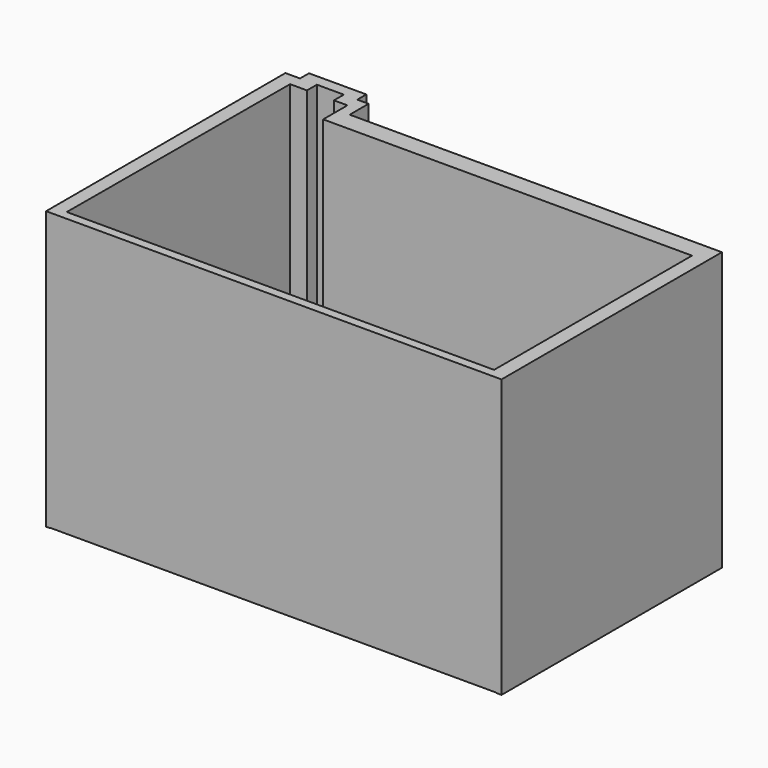
from build123d import *

# Parameters (mm, degrees)
F1_DEPTH      = 50
F2_DEPTH      = 25.4
F4_T1_DEPTH   = 7.325630635
F4_T3_DEPTH   = 9.8896528584
F4_T5_DEPTH   = 10.1948919696
F4_T7_DEPTH   = 14.7742944759
F4_T9_DEPTH   = 106.6527421576
F4_T11_DEPTH  = 67.1516433358
F4_T16_DEPTH  = 88.4586156969
F4_T22_DEPTH  = 17.6426691914
F4_T27_DEPTH  = 122.521271835
F4_T33_DEPTH  = 88.4586156969
F4_T38_DEPTH  = 122.521271835
F4_T47_DEPTH  = 88.4586156969
F4_T53_DEPTH  = 11.110594402
F4_T61_DEPTH  = 88.4586156969
F4_T66_DEPTH  = 11.110594402
F4_T74_DEPTH  = 13.8577054245
F4_T79_DEPTH  = 9.8896528584
F4_T87_DEPTH  = 9.8896528584
F4_T92_DEPTH  = 13.8577054245
F4_T100_DEPTH = 14.7742944759
F4_T105_DEPTH = 10.1948919696
F4_T113_DEPTH = 73.6837181253
F4_T118_DEPTH = 106.6527421576
F4_T126_DEPTH = 129.0533466244
F4_T132_DEPTH = 73.6837181253


# Not quite as in the source:
# - a fillet or chamfer that OpenCascade refuses, or shapes differently, is made with other operations: its cross-section is extruded or revolved along the edge and cut away or added
# - a feature of the source that left no trace in its solid (it failed there, or was rolled back) is left out


with BuildPart() as f1:
    # F0 (on Top) → F1 (new body)
    with BuildSketch(Plane.XY):
        Polygon((55.5458813906, -34.4724208117), (55.5458813906, 37.8682129085), (-45.4904846847, 37.8682129085), (-45.4904846847, 44.2790202796), (-48.5428348184, 44.2790202796), (-48.5428348184, 47.331366688), (-64.1098022461, 47.331366688), (-64.1098022461, 44.2790202796), (-68.0741816759, 44.2790202796), (-68.0741816759, 37.8682129085), (-68.0741816759, 32.6792225242), (-68.0741816759, -36.9142964482), (55.5458813906, -36.9142964482), align=None)
        Polygon((-48.5428348184, 32.6792225242), (51.5778325498, 32.6792225242), (51.5778325498, -34.4724208117), (-64.4113644958, -34.4724208117), (-64.1098022461, 40.9214422107), (-59.5312826335, 40.9214422107), (-59.5312826335, 44.2790202796), (-52.2056519985, 44.2790202796), (-52.2056519985, 40.9214422107), (-48.5428348184, 40.9214422107), align=None, mode=Mode.SUBTRACT)
    extrude(amount=F1_DEPTH)

    # F0 (on Top) + F1_face (on face) → F2 (join)
    with BuildSketch(Plane.XY):
        Polygon((55.5458813906, -34.4724208117), (55.5458813906, 37.8682129085), (-45.4904846847, 37.8682129085), (-45.4904846847, 44.2790202796), (-48.5428348184, 44.2790202796), (-48.5428348184, 47.331366688), (-64.1098022461, 47.331366688), (-64.1098022461, 44.2790202796), (-68.0741816759, 44.2790202796), (-68.0741816759, 37.8682129085), (-68.0741816759, 32.6792225242), (-68.0741816759, -36.9142964482), (55.5458813906, -36.9142964482), align=None)
        Polygon((-48.5428348184, 32.6792225242), (51.5778325498, 32.6792225242), (51.5778325498, -34.4724208117), (-64.4113644958, -34.4724208117), (-64.1098022461, 40.9214422107), (-59.5312826335, 40.9214422107), (-59.5312826335, 44.2790202796), (-52.2056519985, 44.2790202796), (-52.2056519985, 40.9214422107), (-48.5428348184, 40.9214422107), align=None, mode=Mode.SUBTRACT)
    with BuildSketch(Plane(origin=(-7.1792836418, 9.1982220042, 50), x_dir=(1, 0, 0), z_dir=(0, 0, 1))):
        Polygon((62.7251650324, -46.1125184524), (62.7251650324, 28.6699909043), (-38.3112010429, 28.6699909043), (-38.3112010429, 35.0807982755), (-41.3635511765, 35.0807982755), (-41.3635511765, 38.1331446838), (-56.9305186042, 38.1331446838), (-56.9305186042, 35.0807982755), (-60.8948980341, 35.0807982755), (-60.8948980341, -46.1125184524), align=None)
        Polygon((-56.9305186042, 31.7232202065), (-52.3519989917, 31.7232202065), (-52.3519989917, 35.0807982755), (-45.0263683567, 35.0807982755), (-45.0263683567, 31.7232202065), (-41.3635511765, 31.7232202065), (-41.3635511765, 23.48100052), (58.7571161917, 23.48100052), (58.7571161917, -43.6706428158), (-57.2320808539, -43.6706428158), align=None, mode=Mode.SUBTRACT)
    extrude(amount=F2_DEPTH)

    # F4: chamfer of 2.54 on 10 edges, made by hand

    # F4_s2 → F4_t1 (cut)
    with BuildSketch(Plane.YZ.offset(-59.5312826335)):
        Polygon((44.2790202796, 2.54), (46.8190202796, 0), (44.2790202796, 0), align=None)
    extrude(amount=F4_T1_DEPTH, mode=Mode.SUBTRACT)

    # F4_s4 → F4_t3 (cut)
    with BuildSketch(Plane.XZ.offset(-44.2790202796)):
        Polygon((-59.5312826335, 2.54), (-62.0712826335, 0), (-59.5312826335, 0), align=None)
        Polygon((-52.2056519985, 2.54), (-49.6656519985, 0), (-52.2056519985, 0), align=None)
    extrude(amount=F4_T3_DEPTH, mode=Mode.SUBTRACT)

    # F4_s6 → F4_t5 (cut)
    with BuildSketch(Plane.YZ.offset(-58.737726788)):
        Polygon((40.9214422107, 2.54), (43.4614422107, 0), (40.9214422107, 0), align=None)
    extrude(amount=F4_T5_DEPTH, mode=Mode.SUBTRACT)

    # F4_s8 → F4_t7 (cut)
    with BuildSketch(Plane.XZ.offset(-40.9214422107)):
        Polygon((-48.5428348184, 2.54), (-46.0028348184, 0), (-48.5428348184, 0), align=None)
    extrude(amount=F4_T7_DEPTH, mode=Mode.SUBTRACT)

    # F4_s10 → F4_t9 (cut)
    with BuildSketch(Plane.YZ.offset(-55.0749096078)):
        Polygon((32.6792225242, 2.54), (35.2192225242, 0), (32.6792225242, 0), align=None)
    extrude(amount=F4_T9_DEPTH, mode=Mode.SUBTRACT)

    # F4_s12 → F4_t11 (cut)
    with BuildSketch(Plane.XZ.offset(-32.6792225242)):
        Polygon((51.5778325498, 2.54), (54.1178325498, 0), (51.5778325498, 0), align=None)
    extrude(amount=F4_T11_DEPTH, mode=Mode.SUBTRACT)


with BuildPart() as f4_tool14:
    # F4_s15 → F4_t16 (new body)
    with BuildSketch(Plane(origin=(-0.1650388622, -41.2615219051, 0), x_dir=(0, 0, 1), z_dir=(0.0039997929, 0.9999920008, 0))):
        Polygon((2.54, -64.2729667124), (0, -66.8129667124), (0, -64.2729667124), align=None)
    extrude(amount=F4_T16_DEPTH)

    split(bisect_by=Plane.XZ.offset(34.4724208117), keep=Keep.BOTTOM)

    split(bisect_by=Plane.XZ.offset(-40.9214422107), keep=Keep.TOP)


with BuildPart() as f1_1:
    add(f1.part)

    # F4_t13: cut F4_tool14
    add(f4_tool14.part, mode=Mode.SUBTRACT)


with BuildPart() as f4_tool20:
    # F4_s21 → F4_t22 (new body)
    with BuildSketch(Plane.YZ.offset(-70.6418770355)):
        Polygon((40.9214422107, 2.54), (43.4614422107, 0), (40.9214422107, 0), align=None)
    extrude(amount=F4_T22_DEPTH)

    split(bisect_by=Plane(origin=(-64.2724525799, 0.2570785554, 0), x_dir=(0, 0, 1), z_dir=(0.9999920008, -0.0039997929, 0)), keep=Keep.TOP)


with BuildPart() as f1_2:
    add(f1_1.part)

    # F4_t19: cut F4_tool20
    add(f4_tool20.part, mode=Mode.SUBTRACT)


with BuildPart() as f4_tool25:
    # F4_s26 → F4_t27 (new body)
    with BuildSketch(Plane.YZ.offset(51.5778325498)):
        Polygon((-34.4724208117, 2.54), (-37.0124208117, 0), (-34.4724208117, 0), align=None)
    extrude(amount=-F4_T27_DEPTH)

    split(bisect_by=Plane(origin=(-64.2724525799, 0.2570785554, 0), x_dir=(0, 0, 1), z_dir=(0.9999920008, -0.0039997929, 0)), keep=Keep.TOP)


with BuildPart() as f1_3:
    add(f1_2.part)

    # F4_t24: cut F4_tool25
    add(f4_tool25.part, mode=Mode.SUBTRACT)


with BuildPart() as f4_tool31:
    # F4_s32 → F4_t33 (new body)
    with BuildSketch(Plane(origin=(-0.1650388622, -41.2615219051, 0), x_dir=(0, 0, 1), z_dir=(0.0039997929, 0.9999920008, 0))):
        Polygon((2.54, -64.2729667124), (0, -66.8129667124), (0, -64.2729667124), align=None)
    extrude(amount=F4_T33_DEPTH)

    split(bisect_by=Plane.XZ.offset(34.4724208117), keep=Keep.TOP)

    split(bisect_by=Plane.XZ.offset(36.9142964482), keep=Keep.BOTTOM)


with BuildPart() as f4_tool36:
    # F4_s37 → F4_t38 (new body)
    with BuildSketch(Plane.YZ.offset(51.5778325498)):
        Polygon((-34.4724208117, 2.54), (-37.0124208117, 0), (-34.4724208117, 0), align=None)
    extrude(amount=-F4_T38_DEPTH)

    split(bisect_by=Plane(origin=(-64.2724525799, 0.2570785554, 0), x_dir=(0, 0, 1), z_dir=(-0.9999920008, 0.0039997929, 0)), keep=Keep.TOP)

    split(bisect_by=Plane.YZ.offset(-68.0741816759), keep=Keep.TOP)

    split(bisect_by=Plane.XZ.offset(36.9142964482), keep=Keep.BOTTOM)


with BuildPart() as f4_tool31_1:
    add(f4_tool31.part)

    # F4_t42: intersect F4_tool36
    add(f4_tool36.part, mode=Mode.INTERSECT)


with BuildPart() as f1_4:
    add(f1_3.part)

    # F4_t29: cut F4_tool31
    add(f4_tool31_1.part, mode=Mode.SUBTRACT)


with BuildPart() as f4_tool45:
    # F4_s46 → F4_t47 (new body)
    with BuildSketch(Plane(origin=(-0.1650388622, -41.2615219051, 0), x_dir=(0, 0, 1), z_dir=(0.0039997929, 0.9999920008, 0))):
        Polygon((2.54, -64.2729667124), (0, -66.8129667124), (0, -64.2729667124), align=None)
    extrude(amount=F4_T47_DEPTH)

    split(bisect_by=Plane.XZ.offset(-40.9214422107), keep=Keep.BOTTOM)

    split(bisect_by=Plane.XZ.offset(-44.2790202796), keep=Keep.TOP)

    split(bisect_by=Plane.YZ.offset(-64.1098022461), keep=Keep.BOTTOM)


with BuildPart() as f4_tool51:
    # F4_s52 → F4_t53 (new body)
    with BuildSketch(Plane.YZ.offset(-70.6418770355)):
        Polygon((40.9214422107, 2.54), (43.4614422107, 0), (40.9214422107, 0), align=None)
    extrude(amount=F4_T53_DEPTH)

    split(bisect_by=Plane(origin=(-64.2724525799, 0.2570785554, 0), x_dir=(0, 0, 1), z_dir=(-0.9999920008, 0.0039997929, 0)), keep=Keep.TOP)

    split(bisect_by=Plane.YZ.offset(-68.0741816759), keep=Keep.TOP)


with BuildPart() as f4_tool45_1:
    add(f4_tool45.part)

    # F4_t56: intersect F4_tool51
    add(f4_tool51.part, mode=Mode.INTERSECT)


with BuildPart() as f1_5:
    add(f1_4.part)

    # F4_t43: cut F4_tool45
    add(f4_tool45_1.part, mode=Mode.SUBTRACT)


with BuildPart() as f4_tool59:
    # F4_s60 → F4_t61 (new body)
    with BuildSketch(Plane(origin=(-0.1650388622, -41.2615219051, 0), x_dir=(0, 0, 1), z_dir=(0.0039997929, 0.9999920008, 0))):
        Polygon((2.54, -64.2729667124), (0, -66.8129667124), (0, -64.2729667124), align=None)
    extrude(amount=F4_T61_DEPTH)

    split(bisect_by=Plane.XZ.offset(-44.2790202796), keep=Keep.TOP)

    split(bisect_by=Plane.YZ.offset(-64.1098022461), keep=Keep.TOP)


with BuildPart() as f4_tool64:
    # F4_s65 → F4_t66 (new body)
    with BuildSketch(Plane.YZ.offset(-70.6418770355)):
        Polygon((40.9214422107, 2.54), (43.4614422107, 0), (40.9214422107, 0), align=None)
    extrude(amount=F4_T66_DEPTH)

    split(bisect_by=Plane(origin=(-64.2724525799, 0.2570785554, 0), x_dir=(0, 0, 1), z_dir=(-0.9999920008, 0.0039997929, 0)), keep=Keep.TOP)

    split(bisect_by=Plane.YZ.offset(-68.0741816759), keep=Keep.TOP)


with BuildPart() as f4_tool59_1:
    add(f4_tool59.part)

    # F4_t69: intersect F4_tool64
    add(f4_tool64.part, mode=Mode.INTERSECT)


with BuildPart() as f1_6:
    add(f1_5.part)

    # F4_t57: cut F4_tool59
    add(f4_tool59_1.part, mode=Mode.SUBTRACT)


with BuildPart() as f4_tool72:
    # F4_s73 → F4_t74 (new body)
    with BuildSketch(Plane.YZ.offset(-66.063357423)):
        Polygon((44.2790202796, 2.54), (46.8190202796, 0), (44.2790202796, 0), align=None)
    extrude(amount=F4_T74_DEPTH)

    split(bisect_by=Plane.YZ.offset(-59.5312826335), keep=Keep.BOTTOM)

    split(bisect_by=Plane.YZ.offset(-64.1098022461), keep=Keep.TOP)


with BuildPart() as f4_tool77:
    # F4_s78 → F4_t79 (new body)
    with BuildSketch(Plane.XZ.offset(-40.9214422107)):
        Polygon((-59.5312826335, 2.54), (-62.0712826335, 0), (-59.5312826335, 0), align=None)
    extrude(amount=-F4_T79_DEPTH)

    split(bisect_by=Plane.XZ.offset(-44.2790202796), keep=Keep.BOTTOM)

    split(bisect_by=Plane.XZ.offset(-47.331366688), keep=Keep.TOP)


with BuildPart() as f4_tool72_1:
    add(f4_tool72.part)

    # F4_t82: intersect F4_tool77
    add(f4_tool77.part, mode=Mode.INTERSECT)


with BuildPart() as f1_7:
    add(f1_6.part)

    # F4_t70: cut F4_tool72
    add(f4_tool72_1.part, mode=Mode.SUBTRACT)


with BuildPart() as f4_tool85:
    # F4_s86 → F4_t87 (new body)
    with BuildSketch(Plane.XZ.offset(-50.8110950691)):
        Polygon((-52.2056519985, 2.54), (-49.6656519985, 0), (-52.2056519985, 0), align=None)
    extrude(amount=F4_T87_DEPTH)

    split(bisect_by=Plane.XZ.offset(-44.2790202796), keep=Keep.BOTTOM)

    split(bisect_by=Plane.XZ.offset(-47.331366688), keep=Keep.TOP)


with BuildPart() as f4_tool90:
    # F4_s91 → F4_t92 (new body)
    with BuildSketch(Plane.YZ.offset(-59.5312826335)):
        Polygon((44.2790202796, 2.54), (46.8190202796, 0), (44.2790202796, 0), align=None)
    extrude(amount=F4_T92_DEPTH)

    split(bisect_by=Plane.YZ.offset(-52.2056519985), keep=Keep.TOP)

    split(bisect_by=Plane.YZ.offset(-48.5428348184), keep=Keep.BOTTOM)


with BuildPart() as f4_tool85_1:
    add(f4_tool85.part)

    # F4_t95: intersect F4_tool90
    add(f4_tool90.part, mode=Mode.INTERSECT)


with BuildPart() as f1_8:
    add(f1_7.part)

    # F4_t83: cut F4_tool85
    add(f4_tool85_1.part, mode=Mode.SUBTRACT)


with BuildPart() as f4_tool98:
    # F4_s99 → F4_t100 (new body)
    with BuildSketch(Plane.XZ.offset(-47.4535170001)):
        Polygon((-48.5428348184, 2.54), (-46.0028348184, 0), (-48.5428348184, 0), align=None)
    extrude(amount=F4_T100_DEPTH)

    split(bisect_by=Plane.XZ.offset(-40.9214422107), keep=Keep.BOTTOM)

    split(bisect_by=Plane.XZ.offset(-44.2790202796), keep=Keep.TOP)


with BuildPart() as f4_tool103:
    # F4_s104 → F4_t105 (new body)
    with BuildSketch(Plane.YZ.offset(-52.2056519985)):
        Polygon((40.9214422107, 2.54), (43.4614422107, 0), (40.9214422107, 0), align=None)
    extrude(amount=F4_T105_DEPTH)

    split(bisect_by=Plane.YZ.offset(-48.5428348184), keep=Keep.TOP)

    split(bisect_by=Plane.YZ.offset(-45.4904846847), keep=Keep.BOTTOM)


with BuildPart() as f4_tool98_1:
    add(f4_tool98.part)

    # F4_t108: intersect F4_tool103
    add(f4_tool103.part, mode=Mode.INTERSECT)


with BuildPart() as f1_9:
    add(f1_8.part)

    # F4_t96: cut F4_tool98
    add(f4_tool98_1.part, mode=Mode.SUBTRACT)


with BuildPart() as f4_tool111:
    # F4_s112 → F4_t113 (new body)
    with BuildSketch(Plane.XZ.offset(-39.2112973136)):
        Polygon((51.5778325498, 2.54), (54.1178325498, 0), (51.5778325498, 0), align=None)
    extrude(amount=F4_T113_DEPTH)

    split(bisect_by=Plane.XZ.offset(-32.6792225242), keep=Keep.BOTTOM)

    split(bisect_by=Plane.XZ.offset(-37.8682129085), keep=Keep.TOP)


with BuildPart() as f4_tool116:
    # F4_s117 → F4_t118 (new body)
    with BuildSketch(Plane.YZ.offset(-48.5428348184)):
        Polygon((32.6792225242, 2.54), (35.2192225242, 0), (32.6792225242, 0), align=None)
    extrude(amount=F4_T118_DEPTH)

    split(bisect_by=Plane.YZ.offset(55.5458813906), keep=Keep.BOTTOM)

    split(bisect_by=Plane.YZ.offset(51.5778325498), keep=Keep.TOP)


with BuildPart() as f4_tool111_1:
    add(f4_tool111.part)

    # F4_t121: intersect F4_tool116
    add(f4_tool116.part, mode=Mode.INTERSECT)


with BuildPart() as f1_10:
    add(f1_9.part)

    # F4_t109: cut F4_tool111
    add(f4_tool111_1.part, mode=Mode.SUBTRACT)


with BuildPart() as f4_tool124:
    # F4_s125 → F4_t126 (new body)
    with BuildSketch(Plane.YZ.offset(58.1099073392)):
        Polygon((-34.4724208117, 2.54), (-37.0124208117, 0), (-34.4724208117, 0), align=None)
    extrude(amount=-F4_T126_DEPTH)

    split(bisect_by=Plane.YZ.offset(55.5458813906), keep=Keep.BOTTOM)

    split(bisect_by=Plane.YZ.offset(51.5778325498), keep=Keep.TOP)

    split(bisect_by=Plane.XZ.offset(36.9142964482), keep=Keep.BOTTOM)


with BuildPart() as f4_tool130:
    # F4_s131 → F4_t132 (new body)
    with BuildSketch(Plane.XZ.offset(-32.6792225242)):
        Polygon((51.5778325498, 2.54), (54.1178325498, 0), (51.5778325498, 0), align=None)
    extrude(amount=F4_T132_DEPTH)

    split(bisect_by=Plane.XZ.offset(34.4724208117), keep=Keep.TOP)

    split(bisect_by=Plane.XZ.offset(36.9142964482), keep=Keep.BOTTOM)


with BuildPart() as f4_tool124_1:
    add(f4_tool124.part)

    # F4_t135: intersect F4_tool130
    add(f4_tool130.part, mode=Mode.INTERSECT)


with BuildPart() as f1_11:
    add(f1_10.part)

    # F4_t122: cut F4_tool124
    add(f4_tool124_1.part, mode=Mode.SUBTRACT)


solid = f1_11.part
